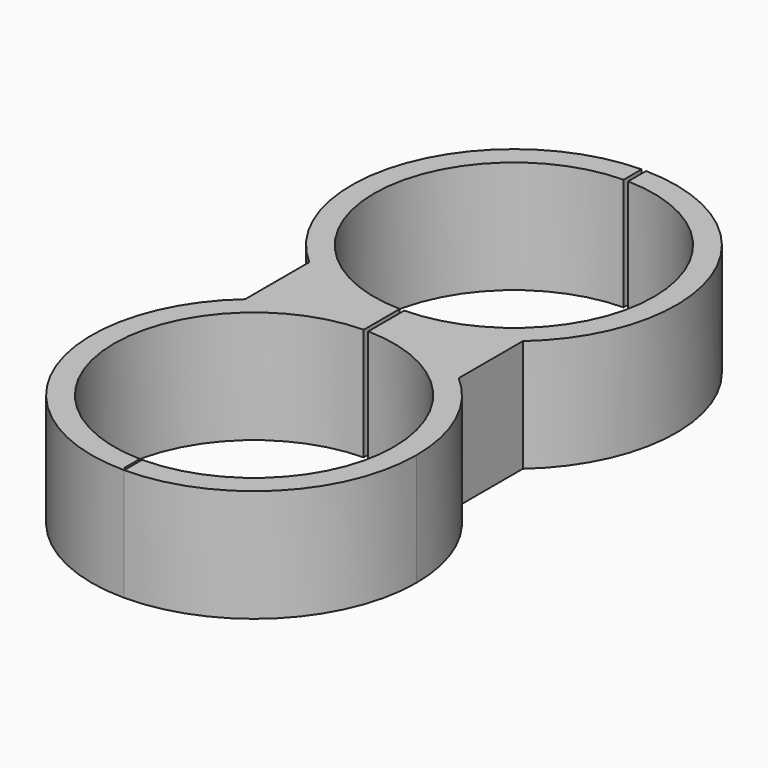
from build123d import *

# Parameters (mm, degrees)
F1_DEPTH = 25


with BuildPart() as f1:
    # F0 (on Top) → F1 (new body)
    with BuildSketch(Plane.XY):
        with BuildLine():
            ThreePointArc((-0.5, -3.905880259), (-31.125, 27.2151034176), (-0.5, 58.3360870942))
            Line((-0.5, 58.3360870942), (-0.5, 63.3366430443))
            ThreePointArc((-0.5, 63.3366430443), (-33.9112453853, 39.6667322838), (-23.756131229, 0))
            ThreePointArc((-23.756131229, 0), (-12.9197959363, -6.5205527634), (-0.5, -8.906436209))
            Line((-0.5, -8.906436209), (-0.5, -3.905880259))
        make_face()
        with BuildLine():
            Line((-0.5, -8.9133569557), (-0.5, -8.906436209))
            ThreePointArc((-0.5, -8.906436209), (-12.9197959363, -6.5205527634), (-23.756131229, 0))
            Line((-23.756131229, 0), (-23.756131229, -17.8197931647))
            ThreePointArc((-23.756131229, -17.8197931647), (-12.9197959363, -11.2992404013), (-0.5, -8.9133569557))
        make_face()
        with BuildLine():
            ThreePointArc((0.5, 58.3360870942), (31.125, 27.2151034176), (0.5, -3.905880259))
            Line((0.5, -3.905880259), (0.5, -8.906436209))
            ThreePointArc((0.5, -8.906436209), (12.9197959363, -6.5205527634), (23.756131229, 0))
            ThreePointArc((23.756131229, 0), (33.9112453853, 39.6667322838), (0.5, 63.3366430443))
            Line((0.5, 63.3366430443), (0.5, 58.3360870942))
        make_face()
        with BuildLine():
            Line((-0.5, -13.9139129058), (-0.5, -8.9133569557))
            ThreePointArc((-0.5, -8.9133569557), (-12.9197959363, -11.2992404013), (-23.756131229, -17.8197931647))
            ThreePointArc((-23.756131229, -17.8197931647), (-33.8242607899, -57.7209127821), (0, -81.1598965824))
            Line((0, -81.1598965824), (0, -80.5474147201))
            Line((0, -80.5474147201), (-0.5, -80.5474147201))
            Line((-0.5, -80.5474147201), (-0.5, -76.155880259))
            ThreePointArc((-0.5, -76.155880259), (-31.125, -45.0348965824), (-0.5, -13.9139129058))
        make_face()
        with BuildLine():
            ThreePointArc((23.756131229, 0), (12.9197959363, -6.5205527634), (0.5, -8.906436209))
            Line((0.5, -8.906436209), (0.5, -8.9133569557))
            ThreePointArc((0.5, -8.9133569557), (12.9197959363, -11.2992404013), (23.756131229, -17.8197931647))
            Line((23.756131229, -17.8197931647), (23.756131229, 0))
        make_face()
        with BuildLine():
            ThreePointArc((23.756131229, -17.8197931647), (12.9197959363, -11.2992404013), (0.5, -8.9133569557))
            Line((0.5, -8.9133569557), (0.5, -13.9139129058))
            ThreePointArc((0.5, -13.9139129058), (22.1847709589, -23.2036904201), (31.125, -45.0348965824))
            ThreePointArc((31.125, -45.0348965824), (22.1847709589, -66.8661027446), (0.5, -76.155880259))
            ThreePointArc((0.5, -76.155880259), (0.2500080653, -76.1588924853), (0, -76.1598965824))
            Line((0, -76.1598965824), (0, -80.5474147201))
            Line((0, -80.5474147201), (0, -81.1598965824))
            ThreePointArc((0, -81.1598965824), (25.5442324704, -70.5791290527), (36.125, -45.0348965824))
            ThreePointArc((36.125, -45.0348965824), (32.8877322542, -30.0879004903), (23.756131229, -17.8197931647))
        make_face()
    extrude(amount=F1_DEPTH)


solid = f1.part
